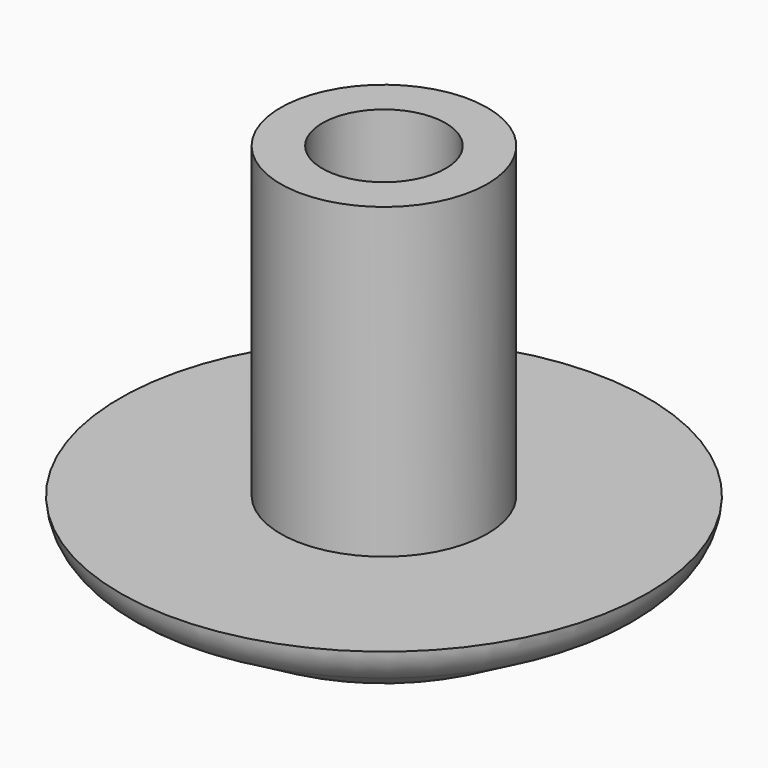
from build123d import *

# Parameters (mm, degrees)
F0_R     = 6
F1_DEPTH = 2
F2_SIZE2 = 2.5980762114
F2_SIZE  = 1.5
F4_R     = 2.35
F4_R_2   = 1.4
F5_DEPTH = 7
F6_R     = 1.2


# Not quite as in the source:
# - a fillet or chamfer that OpenCascade refuses, or shapes differently, is made with other operations: its cross-section is extruded or revolved along the edge and cut away or added


with BuildPart() as f1:
    # F0 (on Top) → F1 (new body)
    with BuildSketch(Plane.XY):
        Circle(F0_R)
    extrude(amount=F1_DEPTH)

    # F2
    f2_edges = [f1.edges().sort_by_distance(p)[0] for p in [
        (-6, 0, 0),
    ]]
    f2_side = f1.faces().sort_by_distance((-6, 0, 1))[0]
    chamfer(f2_edges, length=F2_SIZE, length2=F2_SIZE2, reference=f2_side)

    # F3: fillet of radius 1 on 2 edges, made by hand

    # F3_s1 → F3_t2 (revolve, cut)
    with BuildSketch(Plane.XZ):
        with BuildLine():
            ThreePointArc((3.6339745962, 0.1339745962), (3.3927936413, 0.0340741737), (3.1339745962, 0))
            Line((3.1339745962, 0), (3.4019237886, 0))
            Line((3.4019237886, 0), (3.6339745962, 0.1339745962))
        make_face()
    revolve(axis=Axis((0, 0, 0), (0, 0, 1)), mode=Mode.SUBTRACT)

    # F3_s3 → F3_t4 (revolve, cut)
    with BuildSketch(Plane.XZ):
        with BuildLine():
            ThreePointArc((6, 2), (5.8486778537, 1.5452494356), (5.5031382462, 1.2131367327))
            Line((5.5031382462, 1.2131367327), (6, 1.5))
            Line((6, 1.5), (6, 2))
        make_face()
    revolve(axis=Axis((0, 0, 1.5), (0, 0, 1)), mode=Mode.SUBTRACT)

    # F4 (on face) → F5 (join)
    with BuildSketch(Plane.XY.offset(2)):
        Circle(F4_R)
        Circle(F4_R_2, mode=Mode.SUBTRACT)
    extrude(amount=F5_DEPTH)

    # F6
    f6_edges = [f1.edges().sort_by_distance(p)[0] for p in [
        (-1.4, 0, 2),
    ]]
    fillet(f6_edges, radius=F6_R)


solid = f1.part
